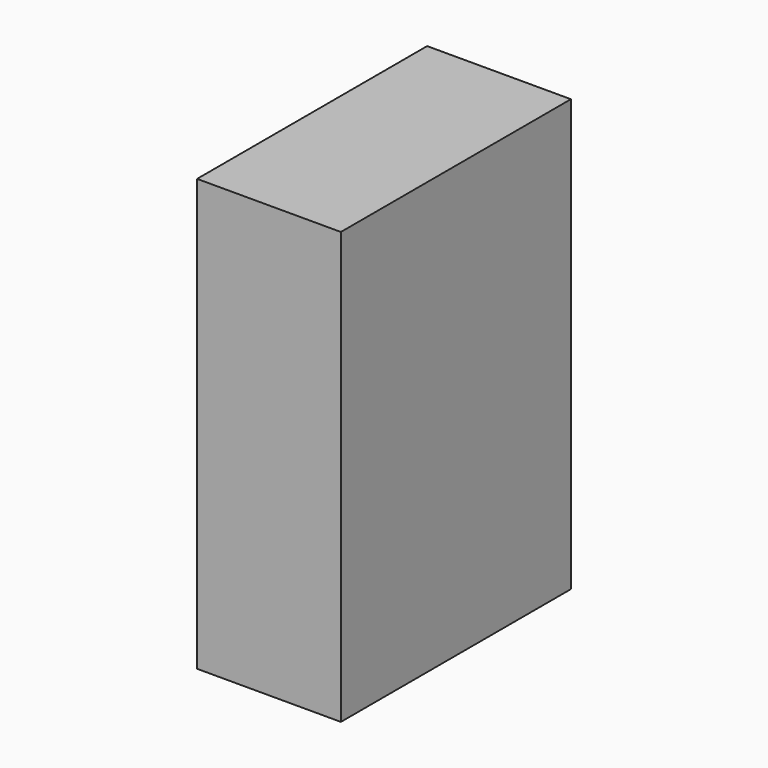
from build123d import *

# Parameters (mm, degrees)
F0_W          = 50
F0_H          = 100
F0_R          = 8.5
F0_R_2        = 5
F0_R_3        = 3.25
F1_DEPTH      = 150
F2_DEPTH      = 100
F3_DEPTH      = 70
F4_DEPTH      = 130
F8_R          = 7.5
F9_DEPTH      = 15
F10_S5_R      = 5
F10_T6_DEPTH  = 12
F10_S11_R     = 5
F10_T12_DEPTH = 12
F10_S17_R     = 5
F10_T18_DEPTH = 12
F11_SIZE      = 8.5


# Not quite as in the source:
# - a fillet or chamfer that OpenCascade refuses, or shapes differently, is made with other operations: its cross-section is extruded or revolved along the edge and cut away or added


with BuildPart() as f1:
    # F0 (on Top) → F1 (new body)
    with BuildSketch(Plane.XY):
        with Locations((25, 50)):
            Rectangle(F0_W, F0_H)
        with Locations((20, 20)):
            Circle(F0_R, mode=Mode.SUBTRACT)
        with Locations((20, 45)):
            Circle(F0_R, mode=Mode.SUBTRACT)
        with Locations((40, 20)):
            Circle(F0_R_2, mode=Mode.SUBTRACT)
        with Locations((40, 45)):
            Circle(F0_R_2, mode=Mode.SUBTRACT)
        with Locations((20, 70)):
            Circle(F0_R, mode=Mode.SUBTRACT)
        with Locations((12.5, 90)):
            Circle(F0_R_3, mode=Mode.SUBTRACT)
        with Locations((40, 70)):
            Circle(F0_R_2, mode=Mode.SUBTRACT)
        with Locations((25, 90)):
            Circle(F0_R_3, mode=Mode.SUBTRACT)
        with Locations((37.5, 90)):
            Circle(F0_R_3, mode=Mode.SUBTRACT)
        with Locations((12.5, 90)):
            Circle(F0_R_3)
        with Locations((25, 90)):
            Circle(F0_R_3)
        with Locations((37.5, 90)):
            Circle(F0_R_3)
        with Locations((40, 70)):
            Circle(F0_R_2)
        with Locations((20, 70)):
            Circle(F0_R)
        with Locations((40, 45)):
            Circle(F0_R_2)
        with Locations((40, 20)):
            Circle(F0_R_2)
        with Locations((20, 20)):
            Circle(F0_R)
        with Locations((20, 45)):
            Circle(F0_R)
    extrude(amount=F1_DEPTH)

    # F0 (on Top) → F2 (cut)
    with BuildSketch(Plane.XY):
        with Locations((20, 20)):
            Circle(F0_R)
        with Locations((20, 45)):
            Circle(F0_R)
        with Locations((20, 70)):
            Circle(F0_R)
    extrude(amount=F2_DEPTH, mode=Mode.SUBTRACT)

    # F0 (on Top) → F3 (cut)
    with BuildSketch(Plane.XY):
        with Locations((37.5, 90)):
            Circle(F0_R_3)
        with Locations((25, 90)):
            Circle(F0_R_3)
        with Locations((12.5, 90)):
            Circle(F0_R_3)
    extrude(amount=F3_DEPTH, mode=Mode.SUBTRACT)

    # F0 (on Top) → F4 (cut)
    with BuildSketch(Plane.XY):
        with Locations((40, 20)):
            Circle(F0_R_2)
        with Locations((40, 45)):
            Circle(F0_R_2)
        with Locations((40, 70)):
            Circle(F0_R_2)
    extrude(amount=F4_DEPTH, mode=Mode.SUBTRACT)

    # F8 (on 3pt) → F9 (cut, symmetric)
    with BuildSketch(Plane.XY.offset(130)):
        with Locations((40, 70)):
            Circle(F8_R)
        with Locations((40, 45)):
            Circle(F8_R)
        with Locations((40, 20)):
            Circle(F8_R)
    extrude(amount=F9_DEPTH, both=True, mode=Mode.SUBTRACT)

    # F10: chamfer of 5 on 3 edges, made by hand


with BuildPart() as f10_tool2:
    # F10_s3 → F10_t4 (revolve)
    with BuildSketch(Plane.XZ.offset(-70)):
        Polygon((42.5, 115), (47.5, 120), (47.5, 115), align=None)
    revolve(axis=Axis((40, 70, 115), (0, 0, 1)))

    # F10_s5 → F10_t6 (cut, symmetric)
    with BuildSketch(Plane.XY.offset(117.5)):
        with Locations((40, 70)):
            Circle(F10_S5_R)
    extrude(amount=F10_T6_DEPTH, both=True, mode=Mode.SUBTRACT)


with BuildPart() as f1_1:
    add(f1.part)

    # F10_t1: union F10_tool2
    add(f10_tool2.part)


with BuildPart() as f10_tool8:
    # F10_s9 → F10_t10 (revolve)
    with BuildSketch(Plane.XZ.offset(-45)):
        Polygon((42.5, 115), (47.5, 120), (47.5, 115), align=None)
    revolve(axis=Axis((40, 45, 115), (0, 0, 1)))

    # F10_s11 → F10_t12 (cut, symmetric)
    with BuildSketch(Plane.XY.offset(117.5)):
        with Locations((40, 45)):
            Circle(F10_S11_R)
    extrude(amount=F10_T12_DEPTH, both=True, mode=Mode.SUBTRACT)


with BuildPart() as f1_2:
    add(f1_1.part)

    # F10_t7: union F10_tool8
    add(f10_tool8.part)


with BuildPart() as f10_tool14:
    # F10_s15 → F10_t16 (revolve)
    with BuildSketch(Plane.XZ.offset(-20)):
        Polygon((42.5, 115), (47.5, 120), (47.5, 115), align=None)
    revolve(axis=Axis((40, 20, 115), (0, 0, 1)))

    # F10_s17 → F10_t18 (cut, symmetric)
    with BuildSketch(Plane.XY.offset(117.5)):
        with Locations((40, 20)):
            Circle(F10_S17_R)
    extrude(amount=F10_T18_DEPTH, both=True, mode=Mode.SUBTRACT)


with BuildPart() as f1_3:
    add(f1_2.part)

    # F10_t13: union F10_tool14
    add(f10_tool14.part)

    # F11
    f11_edges = [f1_3.edges().sort_by_distance(p)[0] for p in [
        (11.5, 70, 100),
        (11.5, 45, 100),
        (11.5, 20, 100),
    ]]
    chamfer(f11_edges, length=F11_SIZE)


solid = f1_3.part
